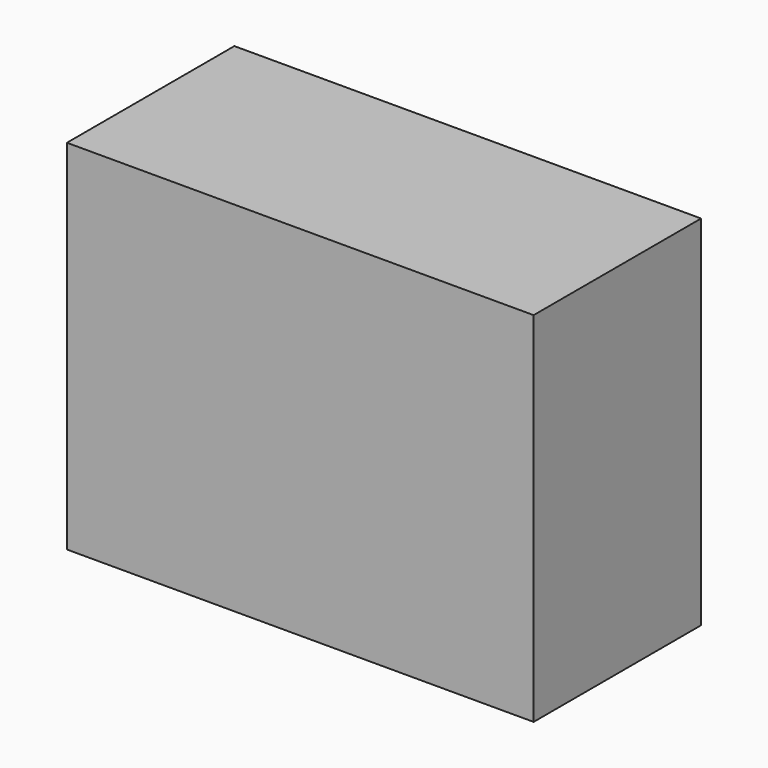
from build123d import *

# Parameters (mm, degrees)
F0_W     = 113.2690608501
F0_H     = 86.9128275663
F2_DEPTH = 25.4
F3_DEPTH = 25.4
F4_T     = -2.54


# Not quite as in the source:
# - a feature names something its author has since deleted; it is built from what else it names
# - the program builds the solid bodies; features that only make, move or delete a surface that nothing else refers to are left out


with BuildPart() as f2:
    # F0 (on Front) → F2 (new body)
    with BuildSketch(Plane.XZ):
        with Locations((-9.0991780162, 12.3919239268)):
            Rectangle(F0_W, F0_H)
    extrude(amount=F2_DEPTH)

    # F3 (add): a face of the model
    f3_faces = [f2.faces().sort_by_distance(p)[0] for p in [
        (-9.0991780162, -25.4, 12.3919239268),
    ]]
    extrude(f3_faces, amount=F3_DEPTH)

    # F4
    f4_openings = [f2.faces().sort_by_distance(p)[0] for p in [
        (-9.099178, 0, 12.391924),
    ]]
    offset(amount=F4_T, openings=f4_openings)


with BuildPart() as f2_1:
    # F10: moved
    add(f2.part)


solid = f2_1.part
